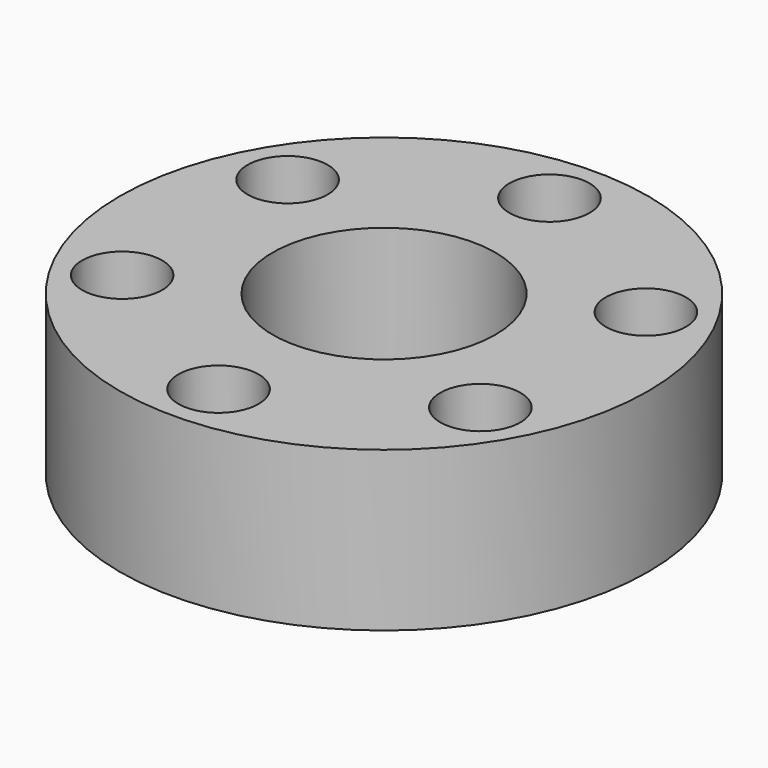
from build123d import *

# Parameters (mm, degrees)
F0_R            = 41.5
F1_DEPTH        = 25
F3_D            = 12.6
F3_COPIES_COUNT = 6
F4_R            = 17.5
F5_DEPTH        = 25.001


# Not quite as in the source:
# - a pattern or mirror of a feature is missing from the dataset's text; its kind, count and spacing are read off the source's solid


with BuildPart() as f1:
    # F0 (on Top) → F1 (new body)
    with BuildSketch(Plane.XY):
        Circle(F0_R)
    extrude(amount=F1_DEPTH)

    # F3 (through all)
    with Locations(Plane.XY.offset(25)):
        with Locations((0, 32.5)):
            f3 = Hole(F3_D / 2)

    # F3_copies: F3 ×6 about axis
    f3_copies_axis = Axis((0, 0, 0), (0, 0, 1))
    for i in range(1, F3_COPIES_COUNT):
        add(f3.rotate(f3_copies_axis, i * 360 / F3_COPIES_COUNT), mode=Mode.SUBTRACT)

    # F4 (on face) → F5 (cut, through all)
    with BuildSketch(Plane.XY.offset(25)):
        Circle(F4_R)
    extrude(amount=-F5_DEPTH, mode=Mode.SUBTRACT)


solid = f1.part
